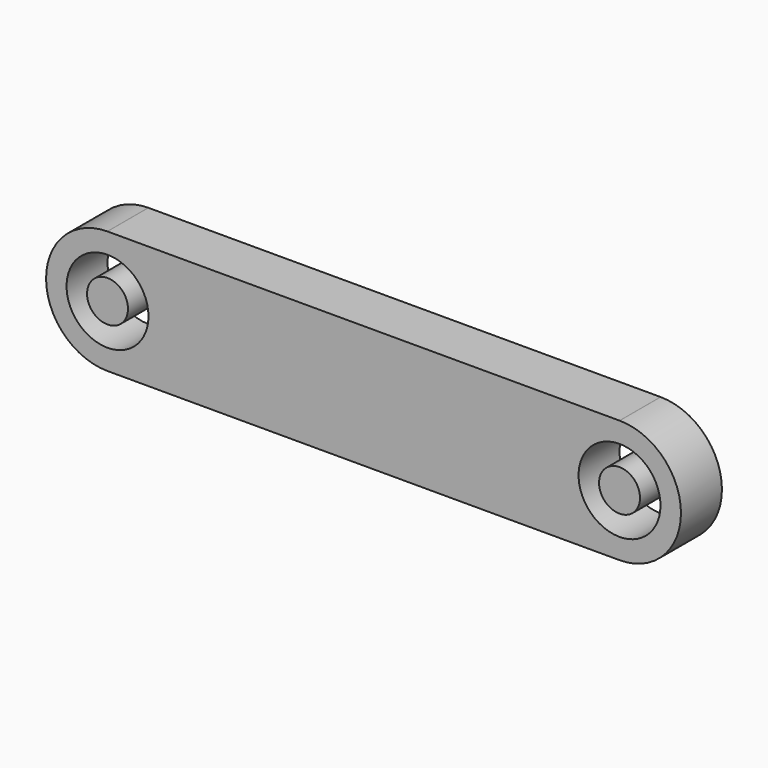
from build123d import *

# Parameters (mm, degrees)
F0_R     = 4
F1_DEPTH = 5
F0_R_2   = 2


# Not quite as in the source:
# - ends of sketch curves that miss each other by under 0.0002 mm in the source are joined


with BuildPart() as f1:
    # F0 (on Front) → F1 (new body)
    with BuildSketch(Plane.XZ):
        with BuildLine():
            Line((0, 6), (-25, 6))
            ThreePointArc((-25, 6), (-25.0125245304, 5.999986928), (-25.0250490062, 5.999947712))
            ThreePointArc((-25.0250490062, 5.999947712), (-30.999986928, -0.0125245304), (-25, -6))
            Line((-25, -6), (0, -6))
            Line((0, -6), (25, -6))
            ThreePointArc((25, -6), (30.999986928, -0.0125245304), (25.0250490062, 5.999947712))
            Line((25.0250490062, 5.999947712), (25, 6))
            Line((25, 6), (0, 6))
        make_face()
        with Locations((-25, 0)):
            Circle(F0_R, mode=Mode.SUBTRACT)
        with Locations((25, 0)):
            Circle(F0_R, mode=Mode.SUBTRACT)
    extrude(amount=F1_DEPTH)


with BuildPart() as f1b:
    # F0 (on Front) → F1, piece 2 (new body)
    with BuildSketch(Plane.XZ):
        with Locations((-25, 0)):
            Circle(F0_R_2)
    extrude(amount=F1_DEPTH)


with BuildPart() as f1c:
    # F0 (on Front) → F1, piece 3 (new body)
    with BuildSketch(Plane.XZ):
        with Locations((25, 0)):
            Circle(F0_R_2)
    extrude(amount=F1_DEPTH)


solid = Compound([f1.part, f1b.part, f1c.part])
